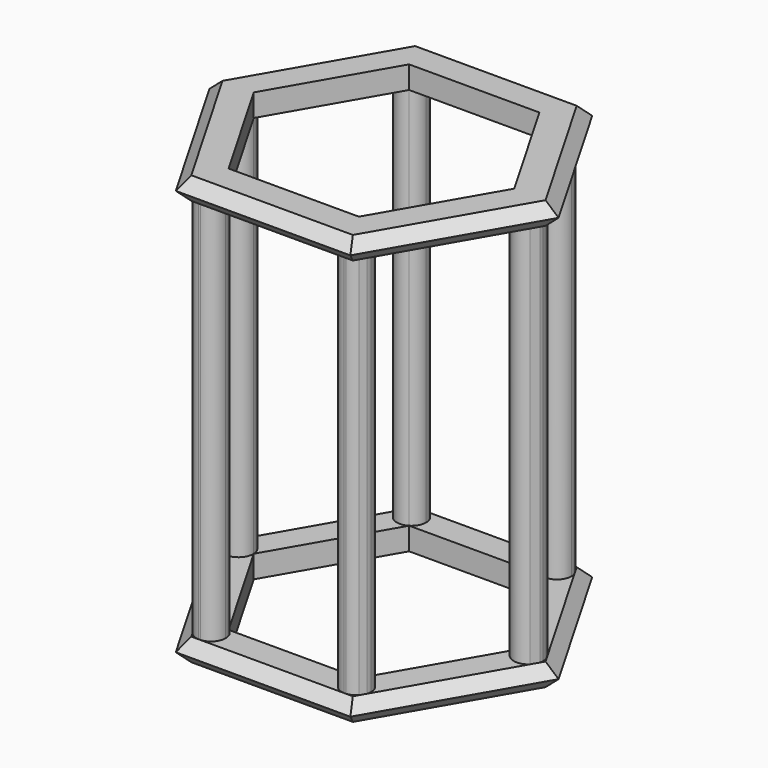
from build123d import *

# Parameters (mm, degrees)
F1_DEPTH     = 6.35
F2_T1_DEPTH  = 77.4547380887
F3_T1_DEPTH  = 71.5888593537
F4_T1_DEPTH  = 71.5888593537
F5_T1_DEPTH  = 71.5888593537
F6_T1_DEPTH  = 71.5888593537
F7_T1_DEPTH  = 65.7229806188
F11_DEPTH    = 6.35
F12_T1_DEPTH = 77.4547380887
F13_T1_DEPTH = 71.5888593537
F14_T1_DEPTH = 71.5888593537
F15_T1_DEPTH = 71.5888593537
F16_T1_DEPTH = 71.5888593537
F17_T1_DEPTH = 65.7229806188
F18_DEPTH    = 107.95


# Not quite as in the source:
# - a fillet or chamfer that OpenCascade refuses, or shapes differently, is made with other operations: its cross-section is extruded or revolved along the edge and cut away or added


with BuildPart() as f1:
    # F0 (on Top) → F1 (new body)
    with BuildSketch(Plane.XY):
        Polygon((25.6632194655, 44.45), (-25.6632194655, 44.45), (-51.326438931, 0), (-25.6632194655, -44.45), (25.6632194655, -44.45), (51.326438931, 0), align=None)
        Polygon((-36.6617420935, 0), (-18.3308710468, 31.75), (18.3308710468, 31.75), (36.6617420935, 0), (18.3308710468, -31.75), (-18.3308710468, -31.75), align=None, mode=Mode.SUBTRACT)
    extrude(amount=F1_DEPTH)

    # F2: chamfer of 5.08 on 2 edges, made by hand

    # F2_s2 → F2_t1 (cut)
    with BuildSketch(Plane.YZ.offset(-38.7273690443)):
        Polygon((-44.45, 5.08), (-39.37, 0), (-44.45, 0), align=None)
        Polygon((-44.45, 1.27), (-39.37, 6.35), (-44.45, 6.35), align=None)
    extrude(amount=F2_T1_DEPTH, mode=Mode.SUBTRACT)

    # F3: chamfer of 5.08 on 2 edges, made by hand

    # F3_s2 → F3_t1 (cut)
    with BuildSketch(Plane(origin=(-16.4307451547, -28.4588854141, 0), x_dir=(0, 0, 1), z_dir=(0.5, 0.8660254038, 0))):
        Polygon((0, 39.37), (5.08, 44.45), (0, 44.45), align=None)
        Polygon((6.35, 39.37), (1.27, 44.45), (6.35, 44.45), align=None)
    extrude(amount=F3_T1_DEPTH, mode=Mode.SUBTRACT)

    # F4: chamfer of 5.08 on 2 edges, made by hand

    # F4_s2 → F4_t1 (cut)
    with BuildSketch(Plane(origin=(16.4307451547, -28.4588854141, 0), x_dir=(0, 0, 1), z_dir=(-0.5, 0.8660254038, 0))):
        Polygon((5.08, 44.45), (0, 39.37), (0, 44.45), align=None)
        Polygon((1.27, 44.45), (6.35, 39.37), (6.35, 44.45), align=None)
    extrude(amount=F4_T1_DEPTH, mode=Mode.SUBTRACT)

    # F5: chamfer of 5.08 on 2 edges, made by hand

    # F5_s2 → F5_t1 (cut)
    with BuildSketch(Plane.YZ.offset(-38.7273690443)):
        Polygon((44.45, 5.08), (39.37, 0), (44.45, 0), align=None)
        Polygon((44.45, 1.27), (39.37, 6.35), (44.45, 6.35), align=None)
    extrude(amount=F5_T1_DEPTH, mode=Mode.SUBTRACT)

    # F6: chamfer of 5.08 on 2 edges, made by hand

    # F6_s2 → F6_t1 (cut)
    with BuildSketch(Plane(origin=(16.4307451547, 28.4588854141, 0), x_dir=(0, 0, 1), z_dir=(-0.5, -0.8660254038, 0))):
        Polygon((0, 39.37), (5.08, 44.45), (0, 44.45), align=None)
        Polygon((1.27, 44.45), (6.35, 39.37), (6.35, 44.45), align=None)
    extrude(amount=F6_T1_DEPTH, mode=Mode.SUBTRACT)

    # F7: chamfer of 5.08 on 2 edges, made by hand

    # F7_s2 → F7_t1 (cut)
    with BuildSketch(Plane(origin=(-16.4307451547, 28.4588854141, 0), x_dir=(0, 0, 1), z_dir=(0.5, -0.8660254038, 0))):
        Polygon((0, 39.37), (5.08, 44.45), (0, 44.45), align=None)
        Polygon((1.27, 44.45), (6.35, 39.37), (6.35, 44.45), align=None)
    extrude(amount=F7_T1_DEPTH, mode=Mode.SUBTRACT)



with BuildPart() as f11:
    # F10 (on offset) → F11 (new body)
    with BuildSketch(Plane(origin=(0, 0, -107.95), x_dir=(1, 0, 0), z_dir=(0, 0, -1))):
        Polygon((25.6632194655, 44.45), (-25.6632194655, 44.45), (-51.326438931, 0), (-25.6632194655, -44.45), (25.6632194655, -44.45), (51.326438931, 0), align=None)
        Polygon((-36.6617420935, 0), (-18.3308710468, 31.75), (18.3308710468, 31.75), (36.6617420935, 0), (18.3308710468, -31.75), (-18.3308710468, -31.75), align=None, mode=Mode.SUBTRACT)
    extrude(amount=F11_DEPTH)

    # F12: chamfer of 5.08 on 2 edges, made by hand

    # F12_s2 → F12_t1 (cut)
    with BuildSketch(Plane(origin=(-19.3636845222, -33.5388854141, 0), x_dir=(0, 0, 1), z_dir=(0.5, 0.8660254038, 0))):
        Polygon((-109.22, -44.45), (-114.3, -39.37), (-114.3, -44.45), align=None)
        Polygon((-113.03, -44.45), (-107.95, -39.37), (-107.95, -44.45), align=None)
    extrude(amount=F12_T1_DEPTH, mode=Mode.SUBTRACT)

    # F13: chamfer of 5.08 on 2 edges, made by hand

    # F13_s2 → F13_t1 (cut)
    with BuildSketch(Plane(origin=(19.3636845222, -33.5388854141, 0), x_dir=(0, 0, 1), z_dir=(-0.5, 0.8660254038, 0))):
        Polygon((-109.22, -44.45), (-114.3, -39.37), (-114.3, -44.45), align=None)
        Polygon((-113.03, -44.45), (-107.95, -39.37), (-107.95, -44.45), align=None)
    extrude(amount=F13_T1_DEPTH, mode=Mode.SUBTRACT)

    # F14: chamfer of 5.08 on 2 edges, made by hand

    # F14_s2 → F14_t1 (cut)
    with BuildSketch(Plane.YZ.offset(-32.8614903094)):
        Polygon((-44.45, -113.03), (-39.37, -107.95), (-44.45, -107.95), align=None)
        Polygon((-44.45, -109.22), (-39.37, -114.3), (-44.45, -114.3), align=None)
    extrude(amount=F14_T1_DEPTH, mode=Mode.SUBTRACT)

    # F15: chamfer of 5.08 on 2 edges, made by hand

    # F15_s2 → F15_t1 (cut)
    with BuildSketch(Plane(origin=(19.3636845222, 33.5388854141, 0), x_dir=(0, 0, 1), z_dir=(-0.5, -0.8660254038, 0))):
        Polygon((-107.95, -39.37), (-113.03, -44.45), (-107.95, -44.45), align=None)
        Polygon((-109.22, -44.45), (-114.3, -39.37), (-114.3, -44.45), align=None)
    extrude(amount=F15_T1_DEPTH, mode=Mode.SUBTRACT)

    # F16: chamfer of 5.08 on 2 edges, made by hand

    # F16_s2 → F16_t1 (cut)
    with BuildSketch(Plane(origin=(-19.3636845222, 33.5388854141, 0), x_dir=(0, 0, 1), z_dir=(0.5, -0.8660254038, 0))):
        Polygon((-107.95, -39.37), (-113.03, -44.45), (-107.95, -44.45), align=None)
        Polygon((-109.22, -44.45), (-114.3, -39.37), (-114.3, -44.45), align=None)
    extrude(amount=F16_T1_DEPTH, mode=Mode.SUBTRACT)

    # F17: chamfer of 5.08 on 2 edges, made by hand

    # F17_s2 → F17_t1 (cut)
    with BuildSketch(Plane.YZ.offset(-32.8614903094)):
        Polygon((39.37, -107.95), (44.45, -113.03), (44.45, -107.95), align=None)
        Polygon((44.45, -109.22), (39.37, -114.3), (44.45, -114.3), align=None)
    extrude(amount=F17_T1_DEPTH, mode=Mode.SUBTRACT)


with BuildPart() as f1_1:
    add(f1.part)

    add(f11.part)  # F18 merges F11
    # F8 (on face) → F18 (join)
    with BuildSketch(Plane(origin=(0, 0, 0), x_dir=(1, 0, 0), z_dir=(0, 0, -1))):
        with BuildLine():
            ThreePointArc((-24.4019218999, 36.4746314671), (-22.996261449, 32.0179739378), (-18.3308710468, 31.75))
            ThreePointArc((-18.3308710468, 31.75), (-16.8828037041, 33.2488412093), (-16.3549710973, 35.2649802766))
            ThreePointArc((-16.3549710973, 35.2649802766), (-17.4635050287, 38.0744368309), (-20.1917663217, 39.37))
            Line((-20.1917663217, 39.37), (-20.7469664852, 39.37))
            ThreePointArc((-20.7469664852, 39.37), (-22.2395757858, 38.9790895208), (-23.4832328124, 38.065847643))
            Line((-23.4832328124, 38.065847643), (-24.4019218999, 36.4746314671))
        make_face()
        with BuildLine():
            ThreePointArc((-44.2711808809, -2.0600654032), (-39.7103407865, -3.8229800416), (-36.6617420935, 0))
            ThreePointArc((-36.6617420935, 0), (-36.6592700651, 0.0824842573), (-36.6584459461, 0.165001434))
            ThreePointArc((-36.6584459461, 0.165001434), (-39.1605946831, 3.9616727057), (-43.6363324768, 3.1596550942))
            Line((-43.6363324768, 3.1596550942), (-44.8066059423, 1.1326819932))
            ThreePointArc((-44.8066059423, 1.1326819932), (-44.8913049977, -0.3338212735), (-44.4575484053, -1.7372673821))
            Line((-44.4575484053, -1.7372673821), (-44.2711808809, -2.0600654032))
        make_face()
        with BuildLine():
            ThreePointArc((20.1917663217, 39.37), (16.4724326672, 36.2410793716), (18.3308710468, 31.75))
            ThreePointArc((18.3308710468, 31.75), (22.4855054708, 31.6784175772), (24.5837617096, 35.2649802766))
            ThreePointArc((24.5837617096, 35.2649802766), (24.5380477999, 35.8766014255), (24.4019218999, 36.4746314671))
            Line((24.4019218999, 36.4746314671), (23.4832328124, 38.065847643))
            ThreePointArc((23.4832328124, 38.065847643), (22.2395757858, 38.9790895208), (20.7469664852, 39.37))
            Line((20.7469664852, 39.37), (20.1917663217, 39.37))
        make_face()
        with BuildLine():
            ThreePointArc((43.6363324768, 3.1596550942), (39.0850907082, 3.9283723543), (36.6617420935, 0))
            ThreePointArc((36.6617420935, 0), (39.7103407865, -3.8229800416), (44.2711808809, -2.0600654032))
            Line((44.2711808809, -2.0600654032), (44.4575484053, -1.7372673821))
            ThreePointArc((44.4575484053, -1.7372673821), (44.8038576253, -0.8140164387), (44.9215282886, 0.165001434))
            ThreePointArc((44.9215282886, 0.165001434), (44.8926971055, 0.6522418291), (44.8066059423, 1.1326819932))
            Line((44.8066059423, 1.1326819932), (43.6363324768, 3.1596550942))
        make_face()
        with BuildLine():
            ThreePointArc((24.5837617096, -35.2649802766), (22.4855054708, -31.6784175772), (18.3308710468, -31.75))
            ThreePointArc((18.3308710468, -31.75), (16.4724326672, -36.2410793716), (20.1917663217, -39.37))
            Line((20.1917663217, -39.37), (20.7469664852, -39.37))
            ThreePointArc((20.7469664852, -39.37), (22.2395757858, -38.9790895208), (23.4832328124, -38.065847643))
            Line((23.4832328124, -38.065847643), (24.4019218999, -36.4746314671))
            ThreePointArc((24.4019218999, -36.4746314671), (24.5380477999, -35.8766014255), (24.5837617096, -35.2649802766))
        make_face()
        with BuildLine():
            ThreePointArc((-16.3549710973, -35.2649802766), (-16.8828037041, -33.2488412093), (-18.3308710468, -31.75))
            ThreePointArc((-18.3308710468, -31.75), (-22.996261449, -32.0179739378), (-24.4019218999, -36.4746314671))
            Line((-24.4019218999, -36.4746314671), (-23.4832328124, -38.065847643))
            ThreePointArc((-23.4832328124, -38.065847643), (-22.2395757858, -38.9790895208), (-20.7469664852, -39.37))
            Line((-20.7469664852, -39.37), (-20.1917663217, -39.37))
            ThreePointArc((-20.1917663217, -39.37), (-17.4635050287, -38.0744368309), (-16.3549710973, -35.2649802766))
        make_face()
    extrude(amount=F18_DEPTH)


solid = f1_1.part
